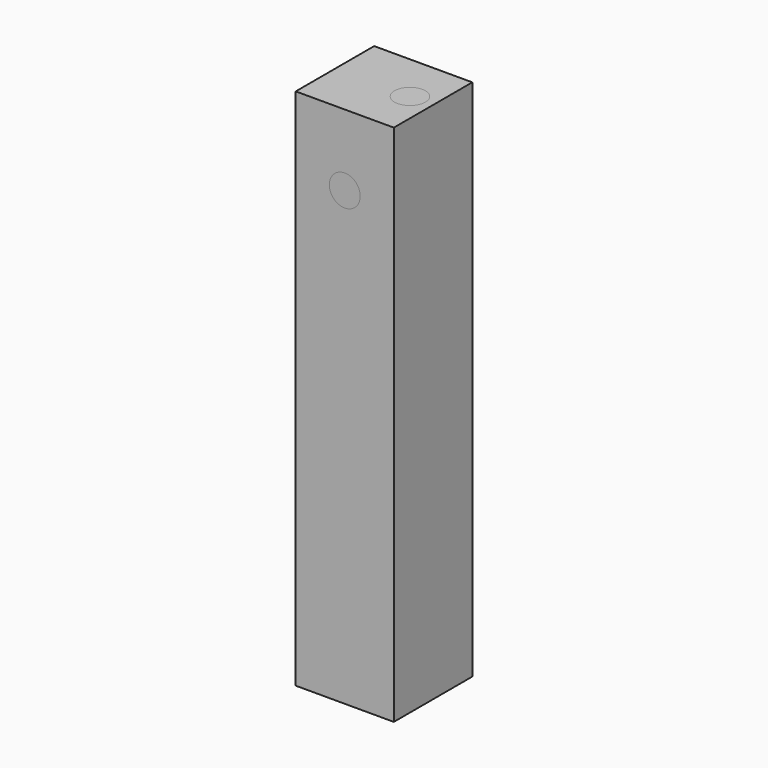
from build123d import *

# Parameters (mm, degrees)
F0_W     = 9.525
F0_H     = 9.525
F1_DEPTH = 50.8
F2_R     = 1.5
F3_DEPTH = 9.525
F4_R     = 2.5
F5_DEPTH = 1
F6_R     = 1.5
F7_DEPTH = 1
F8_R     = 1.5
F9_DEPTH = 12


with BuildPart() as f1:
    # F0 (on Top) → F1 (new body)
    with BuildSketch(Plane.XY):
        with Locations((4.7625, 4.7625)):
            Rectangle(F0_W, F0_H)
    extrude(amount=F1_DEPTH)


with BuildPart() as f3:
    # F2 (on face) → F3 (new body, through all)
    with BuildSketch(Plane(origin=(0, 9.525, 0), x_dir=(-1, 0, 0), z_dir=(0, 1, 0))):
        with Locations((-4.7625, 43.8772141933)):
            Circle(F2_R)
    extrude(amount=-F3_DEPTH)

    # F4 (on face) → F5 (join)
    with BuildSketch(Plane(origin=(0, 9.525, 0), x_dir=(-1, 0, 0), z_dir=(0, 1, 0))):
        with Locations((-4.7625, 43.8772141933)):
            Circle(F4_R)
    extrude(amount=F5_DEPTH)

    # F6 (on face) → F7 (join)
    with BuildSketch(Plane(origin=(0, 10.525, 0), x_dir=(-1, 0, 0), z_dir=(0, 1, 0))):
        with Locations((-4.7625, 43.8772141933)):
            Circle(F6_R)
    extrude(amount=F7_DEPTH)


with BuildPart() as f9:
    # F8 (on face) → F9 (new body)
    with BuildSketch(Plane.XY.offset(50.8)):
        with Locations((7.2815776813, 4.7625)):
            Circle(F8_R)
    extrude(amount=-F9_DEPTH)


solid = Compound([f1.part, f3.part, f9.part])
